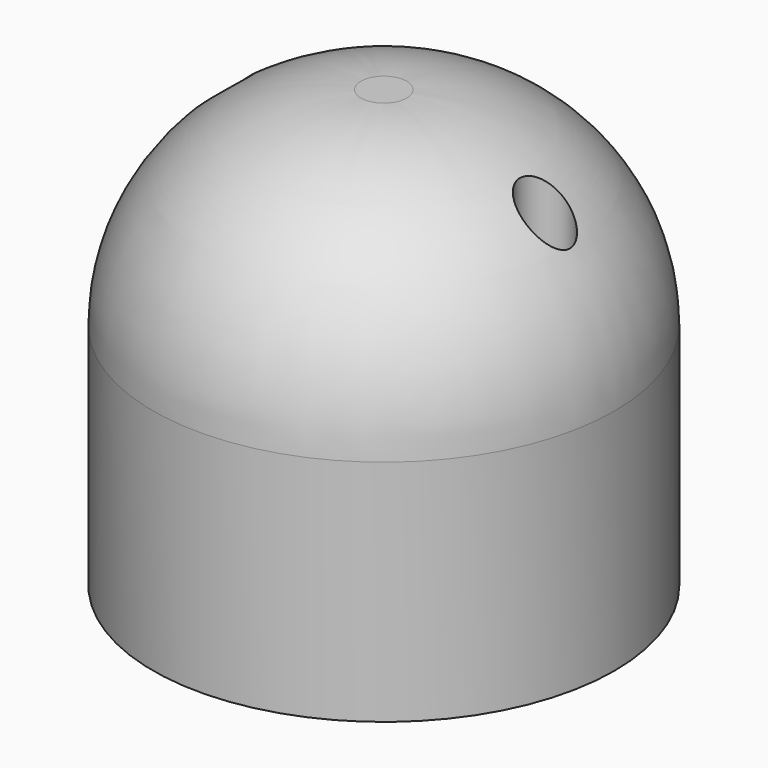
from build123d import *

# Parameters (mm, degrees)
F0_R     = 11.1
F0_R_2   = 1.205
F1_DEPTH = 21


# Not quite as in the source:
# - a fillet or chamfer that OpenCascade refuses, or shapes differently, is made with other operations: its cross-section is extruded or revolved along the edge and cut away or added


with BuildPart() as f1:
    # F0 (on Top) → F1 (new body)
    with BuildSketch(Plane.XY):
        Circle(F0_R)
        with Locations((-7.75, 0)):
            Circle(F0_R_2, mode=Mode.SUBTRACT)
        with Locations((7.75, 0)):
            Circle(F0_R_2, mode=Mode.SUBTRACT)
    extrude(amount=F1_DEPTH)

    # F2: fillet of radius 10 on 1 edges, made by hand

    # F2_s1 → F2_t2 (revolve, cut)
    with BuildSketch(Plane.XZ):
        with BuildLine():
            ThreePointArc((11.1, 11), (8.1710678119, 18.0710678119), (1.1, 21))
            Line((1.1, 21), (11.1, 21))
            Line((11.1, 21), (11.1, 11))
        make_face()
    revolve(axis=Axis((0, 0, 21), (0, 0, 1)), mode=Mode.SUBTRACT)


solid = f1.part
